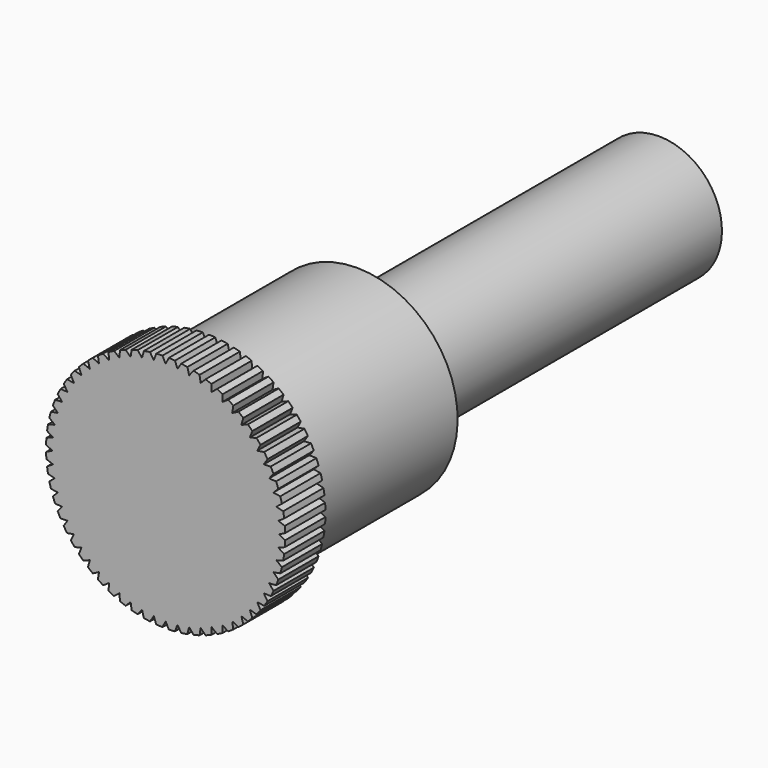
from build123d import *

# Parameters (mm, degrees)
F3_DEPTH        = 4
F3_COPIES_COUNT = 60


# Not quite as in the source:
# - a pattern or mirror of a feature is missing from the dataset's text; its kind, count and spacing are read off the source's solid


with BuildPart() as f1:
    # F0 (on Right) → F1 (revolve)
    with BuildSketch(Plane.YZ):
        Polygon((19, 8), (4, 8), (4, 9.5), (0, 9.5), (0, 0), (19, 0), (49, 0), (49, 5), (19, 5), align=None)
    revolve(axis=Axis((0, -7.8984079883, 0), (0, -1, 0)))

    # F2 (on face) → F3 (cut, through all)
    with BuildSketch(Plane.XZ):
        with BuildLine():
            ThreePointArc((0.25, 9.4967099566), (0, 9.7500216478), (-0.25, 9.4967099566))
            Line((-0.25, 9.4967099566), (0, 9))
            Line((0, 9), (0.25, 9.4967099566))
        make_face()
    f3 = extrude(amount=-F3_DEPTH, mode=Mode.SUBTRACT)

    # F3_copies: F3 ×60 about axis
    f3_copies_axis = Axis((0, 0, 0), (0, 1, 0))
    for i in range(1, F3_COPIES_COUNT):
        add(f3.rotate(f3_copies_axis, i * 360 / F3_COPIES_COUNT), mode=Mode.SUBTRACT)


solid = f1.part
